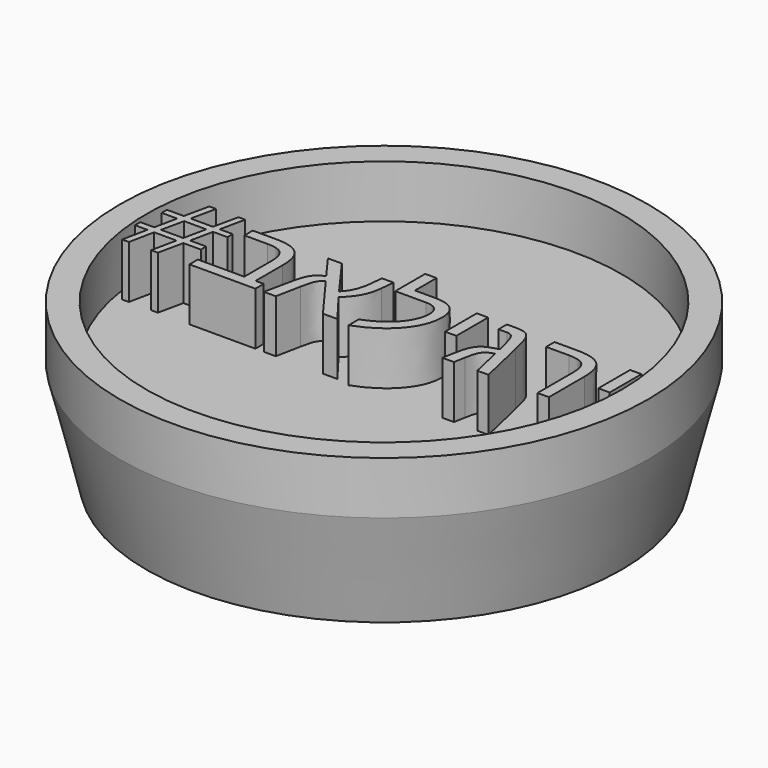
from build123d import *

# Parameters (mm, degrees)
F0_R         = 50
F0_R_2       = 45
F0_TEXT_SIZE = 23.8531652711
F1_DEPTH     = 10
F2_R         = 50
F4_R         = 45


# Not quite as in the source:
# - Text() gives the source's letters only with a copy of the font that has no kerning and outlines rounded to 1/6400 em; it was checked with that copy


with BuildPart() as f1:
    # F0 (on Top) → F1 (new body)
    with BuildSketch(Plane.XY):
        Circle(F0_R)
        Circle(F0_R_2, mode=Mode.SUBTRACT)
        with Locations((-44.1730804365, -8.5871394976)):
            Text('#באליגרי', F0_TEXT_SIZE, font='Arimo', text_align=(TextAlign.LEFT, TextAlign.BOTTOM))
    extrude(amount=F1_DEPTH)


with BuildPart() as f5:
    # F2 (on Top) → F5 section 0
    with BuildSketch(Plane.XY):
        Circle(F2_R)
    # F4 (on offset) → F5 section 1
    with BuildSketch(Plane.XY.offset(-20)):
        Circle(F4_R)
    loft()


solid = Compound([f1.part, f5.part])
